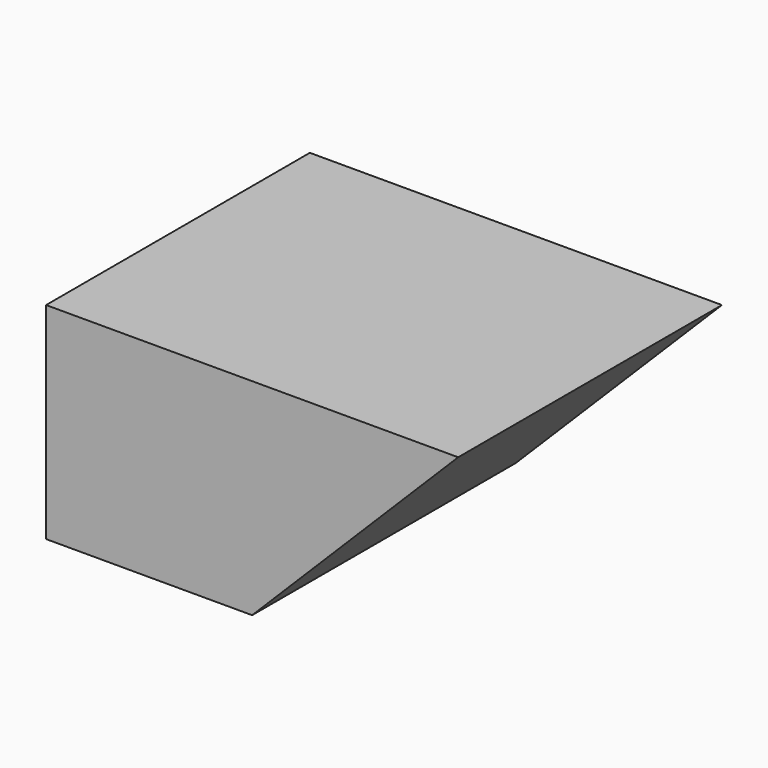
from build123d import *

# Parameters (mm, degrees)
F0_W     = 254
F0_H     = 127
F1_DEPTH = 203.2
F2_SIZE2 = 126.99999
F2_SIZE  = 126.99999


# Not quite as in the source:
# - a fillet or chamfer is up to 0.001 mm smaller than in the source, because OpenCascade refuses the exact size


with BuildPart() as f1:
    # F0 (on Front) → F1 (new body)
    with BuildSketch(Plane.XZ):
        with Locations((-127, 63.5)):
            Rectangle(F0_W, F0_H)
    extrude(amount=F1_DEPTH)

    # F2 (size 127 and 127 in the source; OpenCascade refuses exactly that, so slightly less here)
    f2_edges = [f1.edges().sort_by_distance(p)[0] for p in [
        (0, -101.6, 0),
    ]]
    chamfer(f2_edges, length=F2_SIZE, length2=F2_SIZE2)


solid = f1.part
